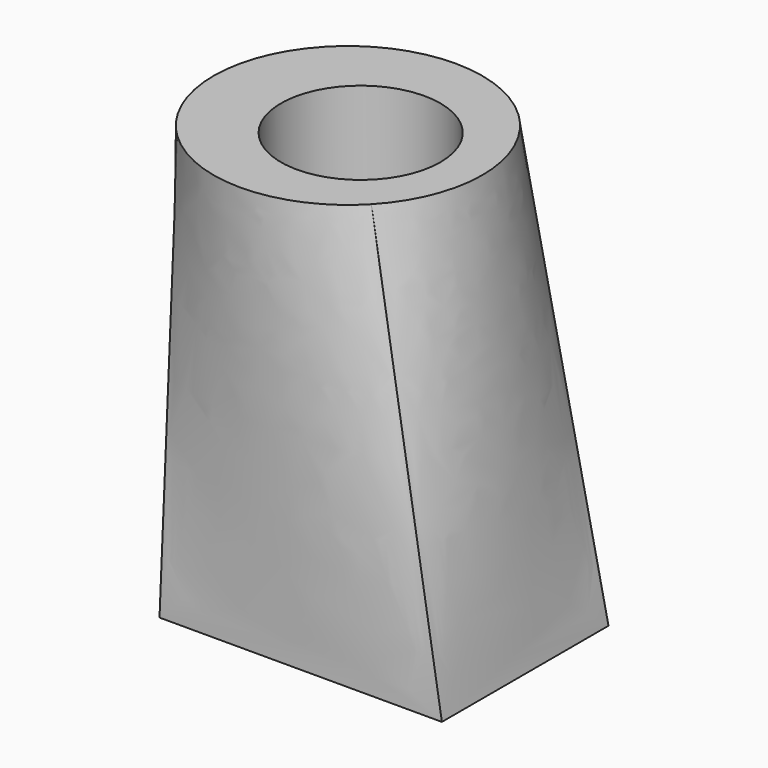
from build123d import *

# Parameters (mm, degrees)
F0_W     = 104.1534732964
F0_H     = 76.8153294921
F4_R     = 29.4148902483
F5_DEPTH = 127


# Not quite as in the source:
# - the arcs of a loft's sections are written as splines that run evenly, so that the points pair up as in the source's solid


with BuildPart() as f3:
    # F0 (on Top) → F3 section 0
    with BuildSketch(Plane.XY):
        with Locations((12.8655565871, 0)):
            Rectangle(F0_W, F0_H)
    # F2 (on offset) → F3 section 1
    with BuildSketch(Plane.XY.offset(152.4)):
        with BuildLine():
            add(Edge.make_bspline(
                [(-41.6450555416, 40.7195541248), (-43.8796016064, 38.3671029534), (-45.8824019296, 35.7946318153), (-49.3477407941, 30.3082562291), (-50.810193648, 27.3944874425), (-53.1386082181, 21.3374769498), (-54.0045123596, 18.1943850152), (-55.1065229691, 11.7995071325), (-55.3426021877, 8.5478793103), (-55.175859187, 2.0608856083), (-54.7730410907, -1.1743198678), (-53.3439523197, -7.5041378591), (-52.3177169821, -10.5985938571), (-49.6812015209, -16.5279847821), (-48.0709865904, -19.3627730932), (-44.3283642496, -24.6638737839), (-42.196049383, -27.1300550832), (-39.8435982116, -29.3646011481)],
                knots=[0, 0, 0, 0, 0.125, 0.125, 0.25, 0.25, 0.375, 0.375, 0.5, 0.5, 0.625, 0.625, 0.75, 0.75, 0.875, 0.875, 1, 1, 1, 1], degree=3))
            add(Edge.make_bspline(
                [(-39.8435982116, -29.3646011481), (-37.4911470402, -31.5991472129), (-34.9186759021, -33.6019475362), (-29.4323003159, -37.0672864006), (-26.5185315293, -38.5297392545), (-20.4615210366, -40.8581538246), (-17.318429102, -41.7240579661), (-10.9235512193, -42.8260685756), (-7.6719233971, -43.0621477942), (-1.1849296951, -42.8954047935), (2.050275781, -42.4925866972), (8.3800937724, -41.0634979262), (11.4745497703, -40.0372625886), (17.4039406953, -37.4007471274), (20.2387290065, -35.7905321969), (25.5398296971, -32.0479098561), (28.0060109965, -29.9155949895), (30.2405570613, -27.5631438181)],
                knots=[0, 0, 0, 0, 0.125, 0.125, 0.25, 0.25, 0.375, 0.375, 0.5, 0.5, 0.625, 0.625, 0.75, 0.75, 0.875, 0.875, 1, 1, 1, 1], degree=3))
            add(Edge.make_bspline(
                [(30.2405570613, -27.5631438181), (32.4751031261, -25.2106926468), (34.4779034494, -22.6382215086), (37.9432423138, -17.1518459224), (39.4056951677, -14.2380771358), (41.7341097378, -8.1810666431), (42.6000138793, -5.0379747085), (43.7020244888, 1.3569031742), (43.9381037074, 4.6085309964), (43.7713607067, 11.0955246984), (43.3685426104, 14.3307301745), (41.9394538394, 20.6605481658), (40.9132185018, 23.7550041638), (38.2767030406, 29.6843950888), (36.6664881101, 32.5191833999), (32.9238657693, 37.8202840906), (30.7915509027, 40.2864653899), (28.4390997313, 42.5210114548)],
                knots=[0, 0, 0, 0, 0.125, 0.125, 0.25, 0.25, 0.375, 0.375, 0.5, 0.5, 0.625, 0.625, 0.75, 0.75, 0.875, 0.875, 1, 1, 1, 1], degree=3))
            add(Edge.make_bspline(
                [(28.4390997313, 42.5210114548), (26.08664856, 44.7555575196), (23.5141774218, 46.7583578429), (18.0278018356, 50.2236967073), (15.114033049, 51.6861495612), (9.0570225563, 54.0145641313), (5.9139306218, 54.8804682728), (-0.480947261, 55.9824788823), (-3.7325750832, 56.2185581009), (-10.2195687852, 56.0518151002), (-13.4547742613, 55.6489970039), (-19.7845922526, 54.2199082329), (-22.8790482506, 53.1936728953), (-28.8084391756, 50.5571574341), (-31.6432274867, 48.9469425036), (-36.9443281774, 45.2043201628), (-39.4105094767, 43.0720052962), (-41.6450555416, 40.7195541248)],
                knots=[0, 0, 0, 0, 0.125, 0.125, 0.25, 0.25, 0.375, 0.375, 0.5, 0.5, 0.625, 0.625, 0.75, 0.75, 0.875, 0.875, 1, 1, 1, 1], degree=3))
        make_face()
    loft(ruled=True)

    # F4 (on face) → F5 (cut)
    with BuildSketch(Plane.XY.offset(152.4)):
        with Locations((0, 5.3224205039)):
            Circle(F4_R)
    extrude(amount=-F5_DEPTH, mode=Mode.SUBTRACT)


solid = f3.part
